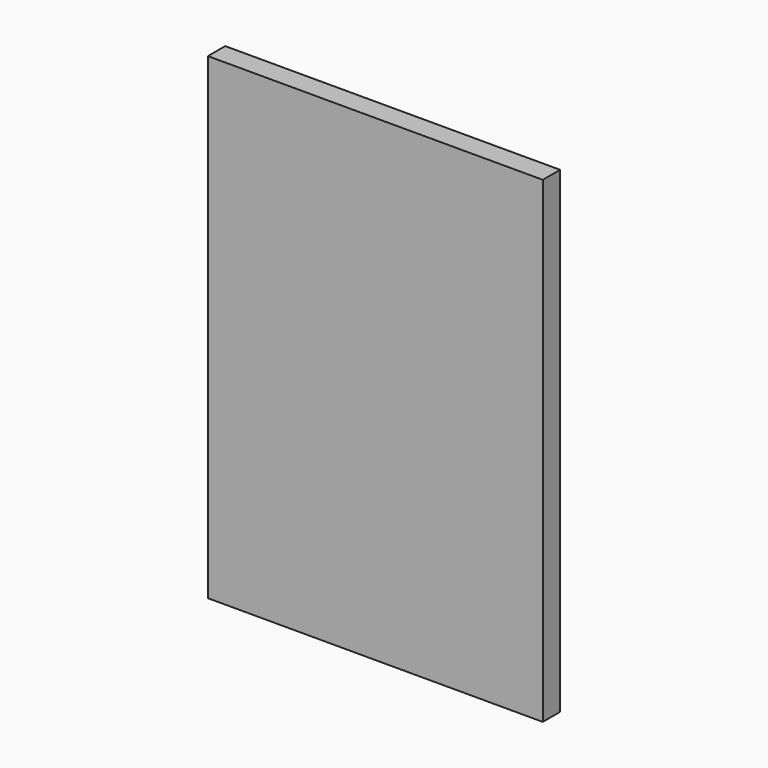
from build123d import *

# Parameters (mm, degrees)
F0_W     = 49.022
F0_H     = 69.85
F1_DEPTH = 3.175


# Not quite as in the source:
# - a length typed as a fraction of an inch, garbled in the dataset ("3 / 203.2 mm" for 3/8 in), is restored


with BuildPart() as f1:
    # F0 (on Front) → F1 (new body)
    with BuildSketch(Plane.XZ):
        with Locations((24.511, 34.925)):
            Rectangle(F0_W, F0_H)
    extrude(amount=F1_DEPTH)


solid = f1.part
